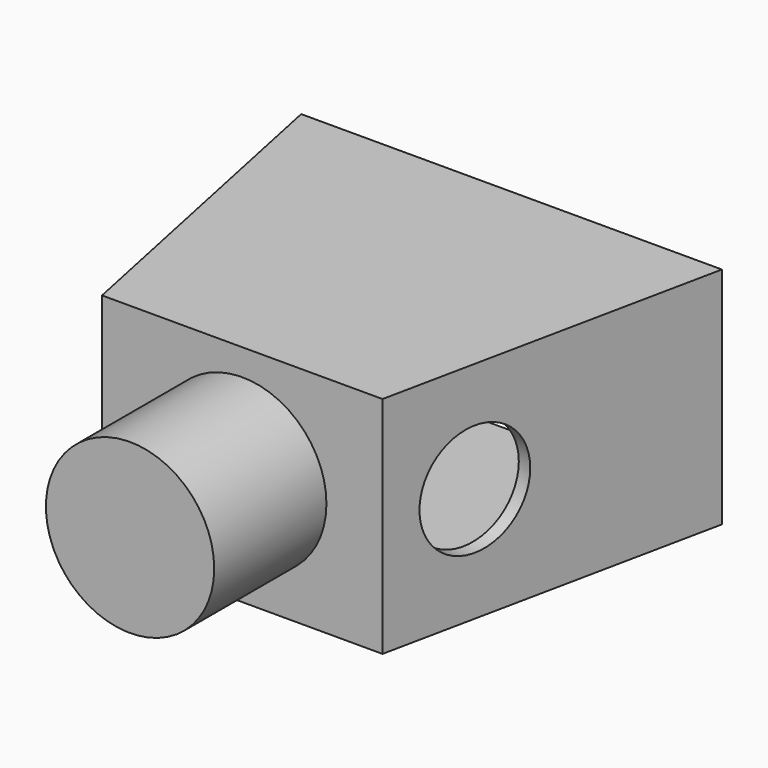
from build123d import *

# Parameters (mm, degrees)
F1_DEPTH = 8
F2_T     = -0.5
F3_R     = 3
F4_DEPTH = 5
F5_R     = 2
F6_DEPTH = 5


# Not quite as in the source:
# - a pattern or mirror of a feature is missing from the dataset's text; its kind, count and spacing are read off the source's solid


with BuildPart() as f1:
    # F0 (on Top) → F1 (new body)
    with BuildSketch(Plane.XY):
        Polygon((-7.5, 0), (-5, -12), (5, -12), (7.5, 0), align=None)
    extrude(amount=F1_DEPTH)

    # F2
    f2_openings = [f1.faces().sort_by_distance(p)[0] for p in [
        (0, 0, 4),
    ]]
    offset(amount=F2_T, openings=f2_openings)

    # F3 (on face) → F4 (join)
    with BuildSketch(Plane.XZ.offset(12)):
        with Locations((0, 4.0601608343)):
            Circle(F3_R)
    extrude(amount=F4_DEPTH)

    # F5 (on face) → F6 (cut)
    with BuildSketch(Plane(origin=(7.1880199667, -1.4975041597, 0), x_dir=(0.2039542541, 0.9789804197, 0), z_dir=(0.9789804197, -0.2039542541, 0))):
        with Locations((-7.3930048384, 4.0684221312)):
            Circle(F5_R)
    f6 = extrude(amount=-F6_DEPTH, mode=Mode.SUBTRACT)

    # F6_copies: F6 across plane
    add(f6.mirror(Plane(origin=(0, 0, 0), x_dir=(0, 0, -1), z_dir=(-1, 0, 0))), mode=Mode.SUBTRACT)


solid = f1.part
